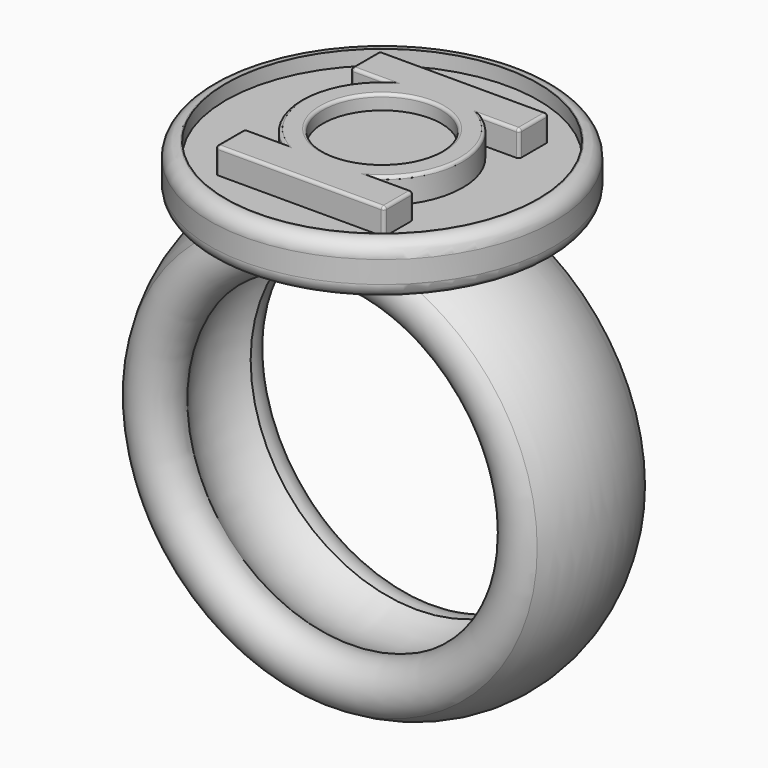
from build123d import *

# Parameters (mm, degrees)
F3_R      = 23.4561334986
F4_DEPTH  = 7
F5_R      = 21.296621693
F6_DEPTH  = 2
F8_DEPTH  = 3.5
F9_R      = 8.0682313044
F10_DEPTH = 2
F11_R     = 2
F12_R     = 0.4


with BuildPart() as f1:
    # F0 (on Top) → F1 (revolve)
    with BuildSketch(Plane.XY):
        with BuildLine():
            ThreePointArc((22.6005557925, 3.1277553644), (24.4153553843, -2.5944045172), (22.1969746053, -8.172522299))
            ThreePointArc((22.1969746053, -8.172522299), (23.8176910174, -12.3691722612), (28.2506942749, -11.6029642522))
            ThreePointArc((28.2506942749, -11.6029642522), (30.9670223358, -2.4214885198), (28.2506942749, 6.7599872127))
            ThreePointArc((28.2506942749, 6.7599872127), (24.2111464827, 6.8330601629), (22.6005557925, 3.1277553644))
        make_face()
    revolve(axis=Axis((0, -1.4125350863, 0), (0, -1, 0)))

    # F3 (on offset) → F4 (join)
    with BuildSketch(Plane.XY.offset(29)):
        with Locations((0, -2.7241741773)):
            Circle(F3_R)
    extrude(amount=F4_DEPTH)

    # F5 (on face) → F6 (cut)
    with BuildSketch(Plane.XY.offset(36)):
        with Locations((0, -2.7241741773)):
            Circle(F5_R)
    extrude(amount=-F6_DEPTH, mode=Mode.SUBTRACT)

    # F7 (on face) → F8 (join)
    with BuildSketch(Plane.XY.offset(34)):
        with BuildLine():
            Line((11.5395749398, 11.2129124999), (-11.4604250602, 11.2129124999))
            Line((-11.4604250602, 11.2129124999), (-11.4604250602, 6.2129124999))
            Line((-11.4604250602, 6.2129124999), (-6.413149127, 6.2129124999))
            ThreePointArc((-6.413149127, 6.2129124999), (-10.9993798942, -2.8409729078), (-6.2219245866, -11.7954284698))
            Line((-6.2219245866, -11.7954284698), (-11.4604250602, -11.7954284698))
            Line((-11.4604250602, -11.7954284698), (-11.4604250602, -16.7954284698))
            Line((-11.4604250602, -16.7954284698), (11.5395749398, -16.7954284698))
            Line((11.5395749398, -16.7954284698), (11.5395749398, -11.7954284698))
            Line((11.5395749398, -11.7954284698), (6.2219245866, -11.7954284698))
            ThreePointArc((6.2219245866, -11.7954284698), (10.9993798942, -2.8409729078), (6.413149127, 6.2129124999))
            Line((6.413149127, 6.2129124999), (11.5395749398, 6.2129124999))
            Line((11.5395749398, 6.2129124999), (11.5395749398, 11.2129124999))
        make_face()
    extrude(amount=F8_DEPTH)

    # F9 (on face) → F10 (cut)
    with BuildSketch(Plane.XY.offset(37.5)):
        with Locations((0, -2.7241741773)):
            Circle(F9_R)
    extrude(amount=-F10_DEPTH, mode=Mode.SUBTRACT)

    # F11
    f11_edges = [f1.edges().sort_by_distance(p)[0] for p in [
        (-23.456133, -2.724174, 29),
        (-23.456133, -2.724174, 36),
    ]]
    fillet(f11_edges, radius=F11_R)

    # F12
    f12_edges = [f1.edges().sort_by_distance(p)[0] for p in [
        (0.039575, -16.795428, 37.5),
        (11.539575, -14.295428, 37.5),
        (8.88075, -11.795428, 37.5),
        (10.99938, -2.840973, 37.5),
        (8.976362, 6.212912, 37.5),
        (11.539575, 8.712912, 37.5),
        (0.039575, 11.212912, 37.5),
        (-11.460425, 8.712912, 37.5),
        (-8.936787, 6.212912, 37.5),
        (-10.99938, -2.840973, 37.5),
        (-8.841175, -11.795428, 37.5),
        (-8.068231, -2.724174, 37.5),
        (-11.460425, -14.295428, 37.5),
        (-11.460425, -16.795428, 35.75),
        (-11.460425, -11.795428, 35.75),
        (-11.460425, 6.212912, 35.75),
        (-11.460425, 11.212912, 35.75),
        (11.539575, 11.212912, 35.75),
        (11.539575, 6.212912, 35.75),
        (11.539575, -16.795428, 35.75),
        (11.539575, -11.795428, 35.75),
    ]]
    fillet(f12_edges, radius=F12_R)


solid = f1.part
